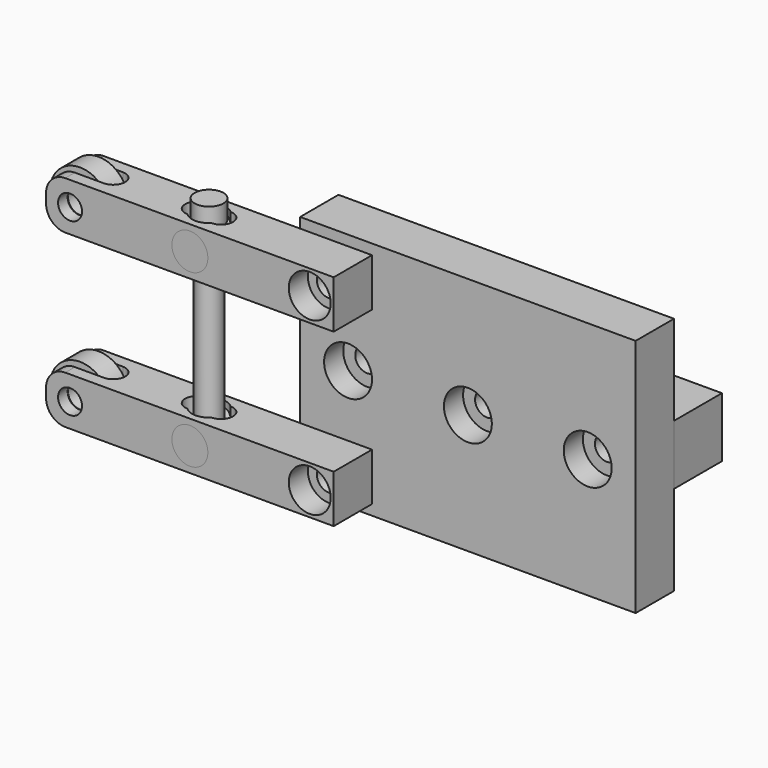
from build123d import *

# Parameters (mm, degrees)
F0_W      = 88.9
F0_H      = 63.5
F0_R      = 3.175
F1_DEPTH  = 6.35
F2_W      = 88.9
F2_H      = 15.875
F2_R      = 3.175
F3_DEPTH  = 15.875
F15_R     = 6.35
F4_DEPTH  = 6.35
F16_W     = 76.2
F16_H     = 12.7
F16_R     = 3.175
F17_DEPTH = 12.7
F5_R      = 5.55625
F18_DEPTH = 6.35
F6_R      = 4.7625
F7_DEPTH  = 12.7
F9_DEPTH  = 60.7795714286
F12_R     = 7.9375
F12_R_2   = 3.175
F20_DEPTH = 3.048
F21_R     = 5.08
F19_R     = 4.7625
F22_DEPTH = 12.7
F13_R     = 3.175
F14_DEPTH = 60.7795714286


# Not quite as in the source:
# - a length typed as a fraction of an inch, garbled in the dataset ("3 / 203.2 mm" for 3/8 in), is restored


with BuildPart() as f1:
    # F0 (on Front) → F1 (new body, symmetric)
    with BuildSketch(Plane.XZ):
        Rectangle(F0_W, F0_H)
        with Locations((-31.75, -22.6785714286)):
            Circle(F0_R, mode=Mode.SUBTRACT)
        with Locations((-31.75, 0)):
            Circle(F0_R, mode=Mode.SUBTRACT)
        with Locations((-31.75, 22.6785714286)):
            Circle(F0_R, mode=Mode.SUBTRACT)
        Circle(F0_R, mode=Mode.SUBTRACT)
        with Locations((31.75, 0)):
            Circle(F0_R, mode=Mode.SUBTRACT)
    extrude(amount=F1_DEPTH, both=True)

    # F15 (on face) → F4 (cut)
    with BuildSketch(Plane.XZ.offset(6.35)):
        with Locations((-31.75, 0)):
            Circle(F15_R)
        Circle(F15_R)
        with Locations((31.75, 0)):
            Circle(F15_R)
    extrude(amount=-F4_DEPTH, mode=Mode.SUBTRACT)


with BuildPart() as f3:
    # F2 (on face) → F3 (new body)
    with BuildSketch(Plane(origin=(0, 6.35, 0), x_dir=(-1, 0, 0), z_dir=(0, 1, 0))):
        Rectangle(F2_W, F2_H)
        with Locations((-31.75, 0)):
            Circle(F2_R, mode=Mode.SUBTRACT)
        Circle(F2_R, mode=Mode.SUBTRACT)
        with Locations((31.75, 0)):
            Circle(F2_R, mode=Mode.SUBTRACT)
    extrude(amount=F3_DEPTH)


with BuildPart() as f17:
    # F16 (on face) → F17 (new body)
    with BuildSketch(Plane.XZ.offset(6.35)):
        with Locations((-63.5, 22.6785714286)):
            Rectangle(F16_W, F16_H)
        with Locations((-95.25, 22.6785714286)):
            Circle(F16_R, mode=Mode.SUBTRACT)
        with Locations((-31.75, 22.6785714286)):
            Circle(F16_R, mode=Mode.SUBTRACT)
    extrude(amount=F17_DEPTH)

    # F5 (on face) → F18 (cut)
    with BuildSketch(Plane.XZ.offset(19.05)):
        with Locations((-31.75, 22.6785714286)):
            Circle(F5_R)
    extrude(amount=-F18_DEPTH, mode=Mode.SUBTRACT)

    # F6 (on face) → F7 (cut, through all)
    with BuildSketch(Plane.XZ.offset(19.05)):
        with Locations((-63.5, 22.6785714286)):
            Circle(F6_R)
    extrude(amount=-F7_DEPTH, mode=Mode.SUBTRACT)

    # F8 (on face) → F9 (cut, through all)
    with BuildSketch(Plane.XY.offset(29.0285714286)):
        with BuildLine():
            Line((-101.6, -15.875), (-88.9, -15.875))
            ThreePointArc((-88.9, -15.875), (-85.725, -12.7), (-88.9, -9.525))
            Line((-88.9, -9.525), (-101.6, -9.525))
            Line((-101.6, -9.525), (-101.6, -15.875))
        make_face()
        with BuildLine():
            ThreePointArc((-66.675, -9.525), (-69.85, -12.7), (-66.675, -15.875))
            ThreePointArc((-66.675, -15.875), (-63.5, -17.1901280605), (-60.325, -15.875))
            ThreePointArc((-60.325, -15.875), (-57.15, -12.7), (-60.325, -9.525))
            ThreePointArc((-60.325, -9.525), (-63.5, -8.2098719395), (-66.675, -9.525))
        make_face()
    extrude(amount=-F9_DEPTH, mode=Mode.SUBTRACT)

    # F21
    f21_edges = [f17.edges().sort_by_distance(p)[0] for p in [
        (-101.6, -17.4625, 29.028571),
        (-101.6, -7.9375, 29.028571),
        (-101.6, -17.4625, 16.328571),
        (-101.6, -7.9375, 16.328571),
    ]]
    fillet(f21_edges, radius=F21_R)


with BuildPart() as f20:
    # F12 (on mid) → F20 (new body, symmetric)
    with BuildSketch(Plane.XZ.offset(12.7)):
        with Locations((-95.25, 22.6785714286)):
            Circle(F12_R)
        with Locations((-95.25, 22.6785714286)):
            Circle(F12_R_2, mode=Mode.SUBTRACT)
    extrude(amount=F20_DEPTH, both=True)


with BuildPart() as f22:
    # F19 (on face) → F22 (new body, through all)
    with BuildSketch(Plane.XZ.offset(19.05)):
        with Locations((-63.5, 22.6785714286)):
            Circle(F19_R)
    extrude(amount=-F22_DEPTH)

    # F13 (on face) → F14 (cut, through all)
    with BuildSketch(Plane.XY.offset(29.0285714286)):
        with Locations((-63.5, -12.7)):
            Circle(F13_R)
    extrude(amount=-F14_DEPTH, mode=Mode.SUBTRACT)


with BuildPart() as f23_1:
    # F23: instance of F20
    add(f20.part.mirror(Plane.XY))


with BuildPart() as f23_2:
    # F23: instance of F17
    add(f17.part.mirror(Plane.XY))


with BuildPart() as f23_3:
    # F23: instance of F22
    add(f22.part.mirror(Plane.XY))


with BuildPart() as f25:
    # F24 (on mid) → F25 (revolve)
    with BuildSketch(Plane.XZ.offset(12.7)):
        Polygon((-59.69, 32.5210714286), (-63.5, 32.5210714286), (-63.5, -27.4410714286), (-60.325, -27.4410714286), (-60.325, 27.4410714286), (-59.69, 27.4410714286), align=None)
    revolve(axis=Axis((-63.5, -12.7, 0), (0, 0, -1)))


solid = Compound([f1.part, f3.part, f17.part, f20.part, f22.part, f23_1.part, f23_2.part, f23_3.part, f25.part])
